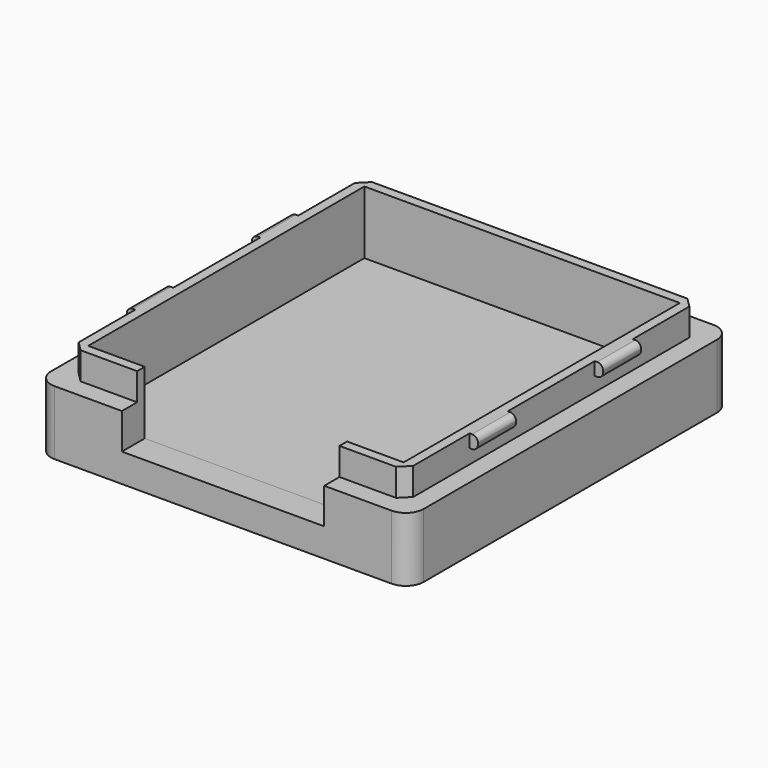
from build123d import *

# Parameters (mm, degrees)
F1_START      = -1
F0_W          = 16
F0_H          = 2.4
F0_W_2        = 2.4
F0_H_2        = 16
F1_DEPTH      = 2.4
F0_W_3        = 31.3
F0_H_3        = 33.8
F2_DEPTH      = 2
F2_DEPTH_BACK = 3.4
F4_W          = 28.1
F4_H          = 30.6
F4_W_2        = 26.5
F4_H_2        = 29
F5_DEPTH      = 2.3
F6_START      = 1.2
F3_W          = 0.8
F3_H          = 4
F3_W_2        = 0.2
F3_W_3        = 0.5
F6_DEPTH      = 0.8
F7_START      = 2
F7_DEPTH      = 2.3
F8_START      = 3.2
F8_DEPTH      = 1.1
F9_R          = 0.5
F11_START     = 14
F10_W         = 17
F10_H         = 7
F11_DEPTH     = 4
F12_R         = 1.5
F14_SIZE      = 0.8


# Not quite as in the source:
# - a feature names something its author has since deleted; it is built from what else it names


with BuildPart() as f1:
    # F0 (on Top) → F1 (new body)
    with BuildSketch(Plane.XY.offset(F1_START)):
        Polygon((-8, 14.5), (-13.25, 14.5), (-13.25, 8), (-10.85, 8), (-10.85, -8), (-13.25, -8), (-13.25, -14.5), (-8, -14.5), (-8, -12.1), (8, -12.1), (8, -14.5), (13.25, -14.5), (13.25, -8), (10.85, -8), (10.85, 8), (13.25, 8), (13.25, 14.5), (8, 14.5), (8, 12.1), (-8, 12.1), align=None)
        with Locations((0, -13.3)):
            Rectangle(F0_W, F0_H)
        with Locations((-12.05, 0)):
            Rectangle(F0_W_2, F0_H_2)
        with Locations((12.05, 0)):
            Rectangle(F0_W_2, F0_H_2)
        with Locations((0, 13.3)):
            Rectangle(F0_W, F0_H)
    extrude(amount=-F1_DEPTH)

    # F0 (on Top) → F2 (join, two sides)
    with BuildSketch(Plane.XY) as f2_sk:
        Rectangle(F0_W_3, F0_H_3)
        Polygon((-13.25, 8), (-13.25, 14.5), (-8, 14.5), (8, 14.5), (13.25, 14.5), (13.25, 8), (13.25, -8), (13.25, -14.5), (8, -14.5), (-8, -14.5), (-13.25, -14.5), (-13.25, -8), align=None, mode=Mode.SUBTRACT)
    extrude(amount=F2_DEPTH)
    extrude(f2_sk.sketch, amount=-F2_DEPTH_BACK)

    # F4 (on face) → F5 (join)
    with BuildSketch(Plane.XY.offset(2)):
        Rectangle(F4_W, F4_H)
        Rectangle(F4_W_2, F4_H_2, mode=Mode.SUBTRACT)
    extrude(amount=F5_DEPTH)

    # F3 (on Top) → F6 (join)
    with BuildSketch(Plane.XY.offset(F6_START)):
        with Locations((-13.6500000894, 6.5681297779)):
            Rectangle(F3_W, F3_H)
        with Locations((-14.1500000894, 6.5681297779)):
            Rectangle(F3_W_2, F3_H)
        with Locations((-14.5000000894, 6.5681297779)):
            Rectangle(F3_W_3, F3_H)
        with Locations((13.6499995038, 6.5681299639)):
            Rectangle(F3_W, F3_H)
        with Locations((14.1499995038, 6.5681299639)):
            Rectangle(F3_W_2, F3_H)
        with Locations((14.4999995038, 6.5681299639)):
            Rectangle(F3_W_3, F3_H)
        with Locations((-14.1500000894, -6.5681295022)):
            Rectangle(F3_W_2, F3_H)
        with Locations((-14.5000000894, -6.5681295022)):
            Rectangle(F3_W_3, F3_H)
        with Locations((-13.6500000894, -6.5681295022)):
            Rectangle(F3_W, F3_H)
        with Locations((14.1499995038, -6.5681295022)):
            Rectangle(F3_W_2, F3_H)
        with Locations((14.4999995038, -6.5681295022)):
            Rectangle(F3_W_3, F3_H)
        with Locations((13.6499995038, -6.5681295022)):
            Rectangle(F3_W, F3_H)
    extrude(amount=F6_DEPTH)

    # F3 (on Top) → F7 (join)
    with BuildSketch(Plane.XY.offset(F7_START)):
        with Locations((-13.6500000894, -6.5681295022)):
            Rectangle(F3_W, F3_H)
        with Locations((-13.6500000894, 6.5681297779)):
            Rectangle(F3_W, F3_H)
        with Locations((13.6499995038, -6.5681295022)):
            Rectangle(F3_W, F3_H)
        with Locations((13.6499995038, 6.5681299639)):
            Rectangle(F3_W, F3_H)
    extrude(amount=F7_DEPTH)

    # F3 (on Top) → F8 (join)
    with BuildSketch(Plane.XY.offset(F8_START)):
        with Locations((-14.5000000894, 6.5681297779)):
            Rectangle(F3_W_3, F3_H)
        with Locations((-14.1500000894, 6.5681297779)):
            Rectangle(F3_W_2, F3_H)
        with Locations((-14.5000000894, -6.5681295022)):
            Rectangle(F3_W_3, F3_H)
        with Locations((-14.1500000894, -6.5681295022)):
            Rectangle(F3_W_2, F3_H)
        with Locations((14.4999995038, 6.5681299639)):
            Rectangle(F3_W_3, F3_H)
        with Locations((14.1499995038, 6.5681299639)):
            Rectangle(F3_W_2, F3_H)
        with Locations((14.4999995038, -6.5681295022)):
            Rectangle(F3_W_3, F3_H)
        with Locations((14.1499995038, -6.5681295022)):
            Rectangle(F3_W_2, F3_H)
    extrude(amount=F8_DEPTH)

    # F9
    f9_edges = [f1.edges().sort_by_distance(p)[0] for p in [
        (13.25, 6.56813, 1.2),
        (14.75, 6.56813, 3.2),
        (-14.75, 6.56813, 3.2),
        (-14.75, 6.56813, 4.3),
        (14.75, -6.56813, 4.3),
        (14.75, -6.56813, 3.2),
        (13.25, -6.56813, 1.2),
        (-14.75, -6.56813, 4.3),
        (-14.75, -6.56813, 3.2),
        (14.75, 6.56813, 4.3),
    ]]
    fillet(f9_edges, radius=F9_R)

    # F10 (on Front) → F11 (cut)
    with BuildSketch(Plane.XZ.offset(F11_START)):
        with Locations((-4.619e-07, 2.5000009835)):
            Rectangle(F10_W, F10_H)
    extrude(amount=F11_DEPTH, mode=Mode.SUBTRACT)

    # F12
    f12_edges = [f1.edges().sort_by_distance(p)[0] for p in [
        (15.65, -16.9, -0.7),
        (15.65, 16.9, -0.7),
        (-15.65, 16.9, -0.7),
        (-15.65, -16.9, -0.7),
    ]]
    fillet(f12_edges, radius=F12_R)

    # F14
    f14_edges = [f1.edges().sort_by_distance(p)[0] for p in [
        (-14.05, 15.3, 3.15),
        (14.05, 15.3, 3.15),
        (-14.05, -15.3, 3.15),
        (14.05, -15.3, 3.15),
    ]]
    chamfer(f14_edges, length=F14_SIZE)


solid = f1.part
